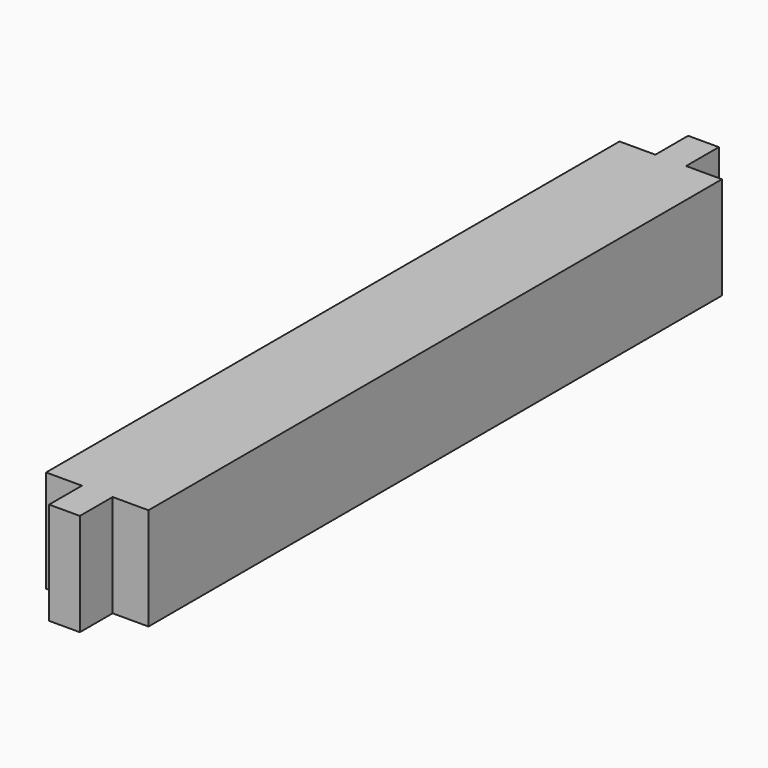
from build123d import *

# Parameters (mm, degrees)
F2_W     = 100
F2_H     = 100
F3_DEPTH = 350
F4_W     = 30
F4_H     = 100
F5_DEPTH = 40


# Not quite as in the source:
# - a pattern or mirror of a feature is missing from the dataset's text; its kind, count and spacing are read off the source's solid


with BuildPart() as f3:
    # F2 (on Front) → F3 (new body, symmetric)
    with BuildSketch(Plane.XZ):
        Rectangle(F2_W, F2_H)
    extrude(amount=F3_DEPTH, both=True)

    # F4 (on face) → F5 (join)
    with BuildSketch(Plane.XZ.offset(350)):
        Rectangle(F4_W, F4_H)
    f5 = extrude(amount=F5_DEPTH)

    # F5_copies: F5 across plane
    add(f5.mirror(Plane.ZX))


solid = f3.part
